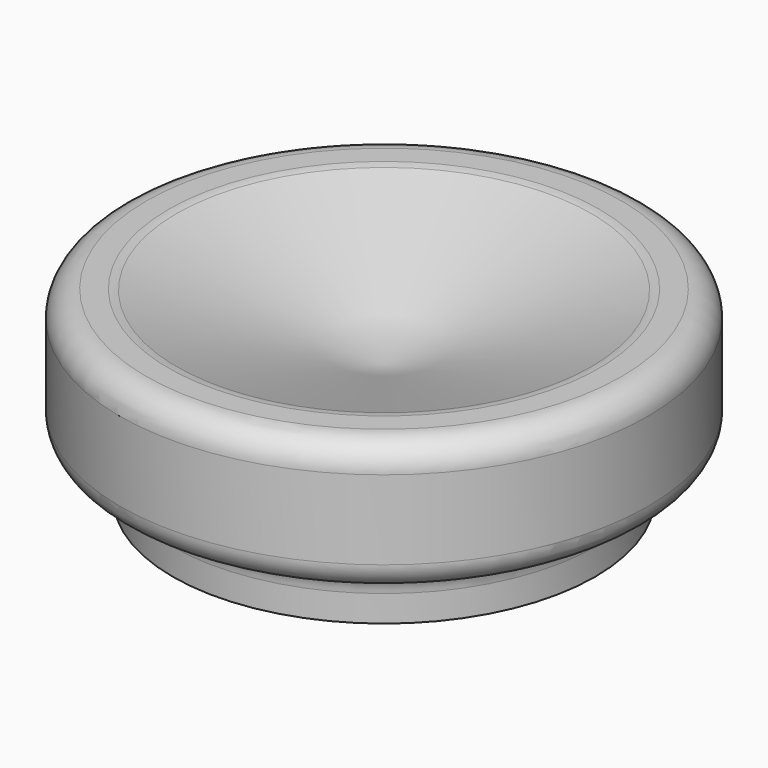
from build123d import *

# Parameters (mm, degrees)
F0_R     = 10
F1_DEPTH = 5
F4_R     = 8
F5_DEPTH = 2
F6_R     = 0.99999


# Not quite as in the source:
# - a fillet or chamfer is up to 0.001 mm smaller than in the source, because OpenCascade refuses the exact size


with BuildPart() as f1:
    # F0 (on Top) → F1 (new body)
    with BuildSketch(Plane.XY):
        Circle(F0_R)
    extrude(amount=F1_DEPTH)

    # F2 (on Front) → F3 (revolve, cut)
    with BuildSketch(Plane.XZ):
        Polygon((-8, 5), (0, 2.5), (0, 5), align=None)
    revolve(axis=Axis((0, 0, 3.75), (0, 0, -1)), mode=Mode.SUBTRACT)

    # F4 (on face) → F5 (join)
    with BuildSketch(Plane(origin=(0, 0, 0), x_dir=(1, 0, 0), z_dir=(0, 0, -1))):
        Circle(F4_R)
    extrude(amount=F5_DEPTH)

    # F6 (radius 1 in the source; OpenCascade refuses exactly that, so slightly less here)
    f6_edges = [f1.edges().sort_by_distance(p)[0] for p in [
        (-8, 0, 0),
        (-10, 0, 0),
        (-10, 0, 5),
        (8, 0, 5),
    ]]
    fillet(f6_edges, radius=F6_R)


solid = f1.part
